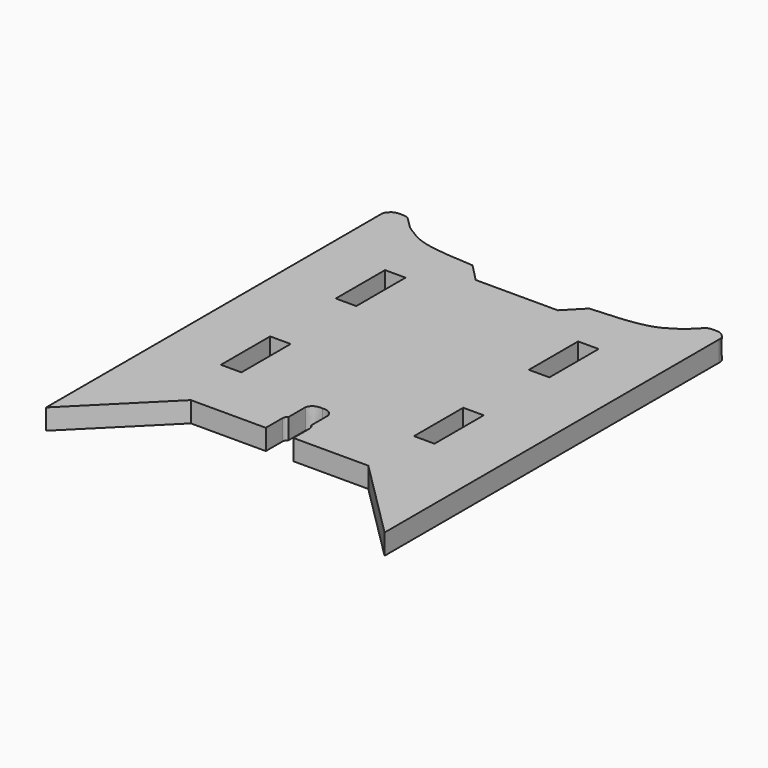
from build123d import *

# Parameters (mm, degrees)
F0_W     = 25.4
F0_H     = 76.2
F1_DEPTH = 25.4


with BuildPart() as f1:
    # F0 (on Top) → F1 (new body)
    with BuildSketch(Plane.XY):
        with BuildLine():
            Line((419.1, 0), (419.1, 29.1582643986))
            Line((419.1, 29.1582643986), (419.1, 517.3072619364))
            add(Edge.make_bspline(
                [(419.1, 517.3072619364), (419.147134559, 518.1974042934), (419.2318387678, 519.7970544265), (418.5736114874, 522.4337537795), (417.4270728627, 524.340815455), (415.824487225, 525.8167119843), (413.4287542387, 528.3993527548), (409.391086273, 530.0033373842), (404.9057722898, 530.0934799636), (398.2767909208, 530.3547825459), (393.7627427273, 528.3669327043), (390.6329406281, 524.4826903766), (386.0666251069, 520.6257581861), (379.3912610246, 512.9725078822), (369.8666381536, 507.866922061), (360.8468497656, 501.5892907558), (346.1541795146, 496.249451646), (324.3776438612, 492.7738532505), (313.0432898306, 492.0475559722), (291.3217386764, 490.4842105973), (280.5920723689, 489.7933052515)],
                knots=[0, 0, 0, 0, 0.0293824295, 0.0595084345, 0.0867094239, 0.1137588548, 0.1481751544, 0.1859995547, 0.2256015417, 0.272993986, 0.3133318288, 0.3535640445, 0.3987236757, 0.4573744575, 0.5181503343, 0.5787543994, 0.6523036094, 0.7362677531, 0.8158837187, 0.8760699048, 0.8760699048, 0.8760699048, 0.8760699048], degree=3))
            Line((280.5920723689, 489.7933052515), (259.2350669765, 467.8874437258))
            Line((259.2350669765, 467.8874437258), (208.4350669765, 467.8874437258))
            Line((208.4350669765, 467.8874437258), (157.6350669765, 467.8874437258))
            Line((157.6350669765, 467.8874437258), (136.0886816558, 489.9119997113))
            add(Edge.make_bspline(
                [(0, 517.3072619364), (-0.047232954, 518.1992624967), (-0.1317917187, 519.7961658976), (0.526377146, 522.4339684383), (1.6729300089, 524.3407612277), (3.2755117734, 525.8167308821), (5.6712460924, 528.3993465881), (9.7089136128, 530.0033391805), (14.1942278227, 530.0934793681), (20.8232087283, 530.3547826623), (25.3372583383, 528.3669327573), (28.4670551881, 524.4826900379), (33.0333949249, 520.6257598555), (39.7086378543, 512.9724994358), (49.233750463, 507.8669545255), (58.2515767921, 501.5891593114), (72.9535489254, 496.2500972756), (94.6899012537, 492.7711419872), (105.9514249536, 492.0689950432), (126.384684191, 490.5612427498), (136.0886816558, 489.9119997113)],
                knots=[0, 0, 0, 0, 0.0294437663, 0.0596326604, 0.0868904328, 0.1139963304, 0.1484844752, 0.1863878353, 0.2260724928, 0.2735638704, 0.3139859199, 0.3543021218, 0.3995560253, 0.4583292427, 0.5192319912, 0.5799625695, 0.6536653159, 0.7378047377, 0.8175869044, 0.8738467686, 0.8738467686, 0.8738467686, 0.8738467686], degree=3))
            Line((0, 517.3072619364), (0, 29.1582643986))
            Line((0, 29.1582643986), (0, 0))
            Line((0, 0), (99.6925341323, 99.4598194957))
            Line((99.6925341323, 99.4598194957), (181.0018675759, 99.4598194957))
            Line((181.0018675759, 99.4598194957), (192.4783936119, 99.4598194957))
            Line((192.4783936119, 99.4598194957), (192.4783936119, 125.5809245631))
            add(Edge.make_bspline(
                [(192.4783936119, 125.5809245631), (192.7145980862, 126.6874069404), (193.1744124211, 128.8413731597), (194.7679380521, 130.1071507729), (195.5428770161, 130.7227043435)],
                knots=[0, 0, 0, 0, 0.5136953251, 1, 1, 1, 1], degree=3))
            Line((195.5428770161, 130.7227043435), (195.5428770161, 157.1194035932))
            add(Edge.make_bspline(
                [(195.5428770161, 157.1194035932), (195.9518024102, 158.2916305791), (196.8054091098, 160.7385825731), (200.1937150151, 163.9060107886), (204.2783832523, 165.573676434), (207.7363179785, 165.5118270656), (209.55, 165.4793871567)],
                knots=[0, 0, 0, 0, 0.2304795373, 0.4811119095, 0.7278439081, 1, 1, 1, 1], degree=3))
            add(Edge.make_bspline(
                [(223.5571229839, 157.1194035932), (223.1481975898, 158.2916305791), (222.2945908902, 160.7385825731), (218.9062849849, 163.9060107886), (214.8216167477, 165.573676434), (211.3636820215, 165.5118270656), (209.55, 165.4793871567)],
                knots=[0, 0, 0, 0, 0.2304795373, 0.4811119095, 0.7278439081, 1, 1, 1, 1], degree=3))
            Line((223.5571229839, 157.1194035932), (223.5571229839, 130.7227043435))
            add(Edge.make_bspline(
                [(226.6216063881, 125.5809245631), (226.3854019138, 126.6874069404), (225.9255875789, 128.8413731597), (224.3320619479, 130.1071507729), (223.5571229839, 130.7227043435)],
                knots=[0, 0, 0, 0, 0.5136953251, 1, 1, 1, 1], degree=3))
            Line((226.6216063881, 125.5809245631), (226.6216063881, 99.4598194957))
            Line((226.6216063881, 99.4598194957), (238.0981324241, 99.4598194957))
            Line((238.0981324241, 99.4598194957), (319.4074658677, 99.4598194957))
            Line((319.4074658677, 99.4598194957), (419.1, 0))
        make_face()
        with Locations((88.9, 213.3992624967)):
            Rectangle(F0_W, F0_H, mode=Mode.SUBTRACT)
        with Locations((327.9701339531, 213.3992624967)):
            Rectangle(F0_W, F0_H, mode=Mode.SUBTRACT)
        with Locations((88.9, 391.1992624967)):
            Rectangle(F0_W, F0_H, mode=Mode.SUBTRACT)
        with Locations((327.9701339531, 391.1992624967)):
            Rectangle(F0_W, F0_H, mode=Mode.SUBTRACT)
    extrude(amount=F1_DEPTH)


solid = f1.part
